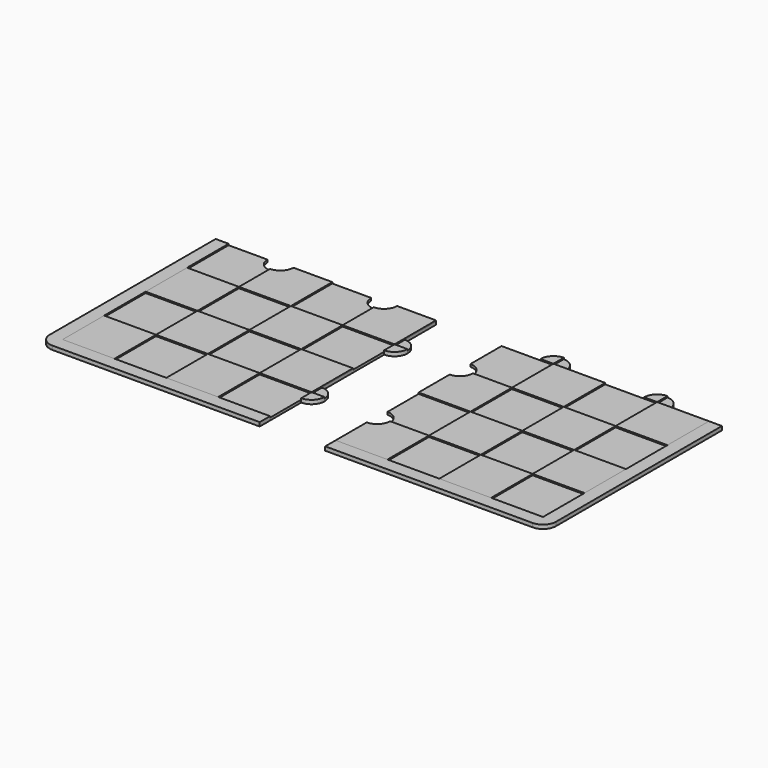
from build123d import *

# Parameters (mm, degrees)
F0_W      = 40
F0_H      = 40
F1_DEPTH  = 2
F3_DEPTH  = 2
F4_DEPTH  = 5
F2_W      = 40
F2_H      = 40
F5_DEPTH  = 1
F6_DEPTH  = 2
F7_DEPTH  = 3
F8_DEPTH  = 4
F9_DEPTH  = 3
F10_DEPTH = 3
F11_DEPTH = 3
F12_DEPTH = 2


with BuildPart() as f1:
    # F0 (on Top) → F1 (new body)
    with BuildSketch(Plane.XY):
        with BuildLine():
            Line((-100, -20), (-60, -20))
            Line((-60, -20), (-60, 10))
            ThreePointArc((-60, 10), (-67.0710678119, 12.9289321881), (-70, 20))
            Line((-70, 20), (-100, 20))
            Line((-100, 20), (-100, -20))
        make_face()
        with BuildLine():
            ThreePointArc((-70, 20), (-67.0710678119, 12.9289321881), (-60, 10))
            Line((-60, 10), (-60, 20))
            Line((-60, 20), (-70, 20))
        make_face()
        with BuildLine():
            ThreePointArc((-60, 10), (-52.9289321881, 12.9289321881), (-50, 20))
            Line((-50, 20), (-60, 20))
            Line((-60, 20), (-60, 10))
        make_face()
        with BuildLine():
            Line((-60, -20), (-20, -20))
            Line((-20, -20), (-20, 20))
            Line((-20, 20), (-50, 20))
            ThreePointArc((-50, 20), (-52.9289321881, 12.9289321881), (-60, 10))
            Line((-60, 10), (-60, -20))
        make_face()
        with BuildLine():
            Line((-20, -20), (20, -20))
            Line((20, -20), (20, 10))
            ThreePointArc((20, 10), (12.9289321881, 12.9289321881), (10, 20))
            Line((10, 20), (-20, 20))
            Line((-20, 20), (-20, -20))
        make_face()
        with BuildLine():
            ThreePointArc((10, 20), (12.9289321881, 12.9289321881), (20, 10))
            Line((20, 10), (20, 20))
            Line((20, 20), (10, 20))
        make_face()
        with BuildLine():
            Line((20, 20), (20, 10))
            ThreePointArc((20, 10), (27.0710678119, 12.9289321881), (30, 20))
            Line((30, 20), (20, 20))
        make_face()
        with BuildLine():
            Line((20, 10), (20, -20))
            Line((20, -20), (50, -20))
            ThreePointArc((50, -20), (52.9289321881, -12.9289321881), (60, -10))
            Line((60, -10), (60, 20))
            Line((60, 20), (30, 20))
            ThreePointArc((30, 20), (27.0710678119, 12.9289321881), (20, 10))
        make_face()
        with BuildLine():
            ThreePointArc((60, -10), (52.9289321881, -12.9289321881), (50, -20))
            Line((50, -20), (60, -20))
            Line((60, -20), (60, -10))
        make_face()
        with BuildLine():
            Line((60, -20), (50, -20))
            ThreePointArc((50, -20), (52.9289321881, -27.0710678119), (60, -30))
            Line((60, -30), (60, -20))
        make_face()
        with BuildLine():
            Line((50, -20), (20, -20))
            Line((20, -20), (20, -60))
            Line((20, -60), (60, -60))
            Line((60, -60), (60, -30))
            ThreePointArc((60, -30), (52.9289321881, -27.0710678119), (50, -20))
        make_face()
        with Locations((0, -40)):
            Rectangle(F0_W, F0_H)
        with Locations((-40, -40)):
            Rectangle(F0_W, F0_H)
        with Locations((-80, -40)):
            Rectangle(F0_W, F0_H)
        with Locations((-80, -80)):
            Rectangle(F0_W, F0_H)
        with BuildLine():
            Line((-60, -140), (-60, -100))
            Line((-60, -100), (-100, -100))
            Line((-100, -100), (-100, -130))
            ThreePointArc((-100, -130), (-92.9289321881, -132.9289321881), (-90, -140))
            Line((-90, -140), (-60, -140))
        make_face()
        with Locations((-40, -120)):
            Rectangle(F0_W, F0_H)
        with Locations((-40, -80)):
            Rectangle(F0_W, F0_H)
        with Locations((0, -80)):
            Rectangle(F0_W, F0_H)
        with Locations((0, -120)):
            Rectangle(F0_W, F0_H)
        with BuildLine():
            Line((50, -100), (20, -100))
            Line((20, -100), (20, -140))
            Line((20, -140), (60, -140))
            Line((60, -140), (60, -110))
            ThreePointArc((60, -110), (52.9289321881, -107.0710678119), (50, -100))
        make_face()
        with BuildLine():
            Line((60, -60), (20, -60))
            Line((20, -60), (20, -100))
            Line((20, -100), (50, -100))
            ThreePointArc((50, -100), (52.9289321881, -92.9289321881), (60, -90))
            Line((60, -90), (60, -60))
        make_face()
        with BuildLine():
            Line((60, -100), (60, -90))
            ThreePointArc((60, -90), (52.9289321881, -92.9289321881), (50, -100))
            Line((50, -100), (60, -100))
        make_face()
        with BuildLine():
            Line((60, -100), (50, -100))
            ThreePointArc((50, -100), (52.9289321881, -107.0710678119), (60, -110))
            Line((60, -110), (60, -100))
        make_face()
        with BuildLine():
            ThreePointArc((-90, -140), (-92.9289321881, -132.9289321881), (-100, -130))
            Line((-100, -130), (-100, -140))
            Line((-100, -140), (-90, -140))
        make_face()
    extrude(amount=F1_DEPTH)

    # F0 (on Top) → F3 (join)
    with BuildSketch(Plane.XY):
        with BuildLine():
            ThreePointArc((70, -100), (67.0710678119, -92.9289321881), (60, -90))
            Line((60, -90), (60, -100))
            Line((60, -100), (70, -100))
        make_face()
        with BuildLine():
            Line((60, -10), (60, -20))
            Line((60, -20), (70, -20))
            ThreePointArc((70, -20), (67.0710678119, -12.9289321881), (60, -10))
        make_face()
    extrude(amount=F3_DEPTH)

    # F0 (on Top) → F4 (cut)
    with BuildSketch(Plane.XY):
        with BuildLine():
            ThreePointArc((-70, 20), (-67.0710678119, 12.9289321881), (-60, 10))
            Line((-60, 10), (-60, 20))
            Line((-60, 20), (-70, 20))
        make_face()
        with BuildLine():
            ThreePointArc((-60, 10), (-52.9289321881, 12.9289321881), (-50, 20))
            Line((-50, 20), (-60, 20))
            Line((-60, 20), (-60, 10))
        make_face()
        with BuildLine():
            ThreePointArc((10, 20), (12.9289321881, 12.9289321881), (20, 10))
            Line((20, 10), (20, 20))
            Line((20, 20), (10, 20))
        make_face()
        with BuildLine():
            Line((20, 20), (20, 10))
            ThreePointArc((20, 10), (27.0710678119, 12.9289321881), (30, 20))
            Line((30, 20), (20, 20))
        make_face()
    extrude(amount=F4_DEPTH, mode=Mode.SUBTRACT)

    # F0 (on Top) → F10 (join)
    with BuildSketch(Plane.XY):
        with BuildLine():
            Line((70, -100), (60, -100))
            Line((60, -100), (60, -110))
            ThreePointArc((60, -110), (67.0710678119, -107.0710678119), (70, -100))
        make_face()
        with BuildLine():
            Line((70, -20), (60, -20))
            Line((60, -20), (60, -30))
            ThreePointArc((60, -30), (67.0710678119, -27.0710678119), (70, -20))
        make_face()
    extrude(amount=F10_DEPTH)


with BuildPart() as f5:
    # F2 (on face) → F5 (new body)
    with BuildSketch(Plane.XY.offset(2)):
        with Locations((-80, -120)):
            Rectangle(F2_W, F2_H)
    extrude(amount=F5_DEPTH)


with BuildPart() as f5b:
    # F2 (on face) → F5, piece 2 (new body)
    with BuildSketch(Plane.XY.offset(2)):
        with Locations((0, -120)):
            Rectangle(F2_W, F2_H)
    extrude(amount=F5_DEPTH)


with BuildPart() as f5c:
    # F2 (on face) → F5, piece 3 (new body)
    with BuildSketch(Plane.XY.offset(2)):
        with Locations((-40, -80)):
            Rectangle(F2_W, F2_H)
    extrude(amount=F5_DEPTH)


with BuildPart() as f5d:
    # F2 (on face) → F5, piece 4 (new body)
    with BuildSketch(Plane.XY.offset(2)):
        with Locations((40, -80)):
            Rectangle(F2_W, F2_H)
    extrude(amount=F5_DEPTH)


with BuildPart() as f5e:
    # F2 (on face) → F5, piece 5 (new body)
    with BuildSketch(Plane.XY.offset(2)):
        with Locations((-80, -40)):
            Rectangle(F2_W, F2_H)
    extrude(amount=F5_DEPTH)


with BuildPart() as f5f:
    # F2 (on face) → F5, piece 6 (new body)
    with BuildSketch(Plane.XY.offset(2)):
        with Locations((0, -40)):
            Rectangle(F2_W, F2_H)
    extrude(amount=F5_DEPTH)


with BuildPart() as f5g:
    # F2 (on face) → F5, piece 7 (new body)
    with BuildSketch(Plane.XY.offset(2)):
        with BuildLine():
            Line((60, -20), (60, 20))
            Line((60, 20), (30, 20))
            ThreePointArc((30, 20), (27.0710678119, 12.9289321881), (20, 10))
            Line((20, 10), (20, -20))
            Line((20, -20), (60, -20))
        make_face()
    extrude(amount=F5_DEPTH)


with BuildPart() as f5h:
    # F2 (on face) → F5, piece 8 (new body)
    with BuildSketch(Plane.XY.offset(2)):
        with BuildLine():
            Line((-60, -20), (-20, -20))
            Line((-20, -20), (-20, 20))
            Line((-20, 20), (-50, 20))
            ThreePointArc((-50, 20), (-52.9289321881, 12.9289321881), (-60, 10))
            Line((-60, 10), (-60, -20))
        make_face()
    extrude(amount=F5_DEPTH)


with BuildPart() as f6:
    # F0 (on Top) → F6 (new body)
    with BuildSketch(Plane.XY):
        with BuildLine():
            Line((150.5487942696, -140), (150.5487942696, -100))
            Line((150.5487942696, -100), (120.5487942696, -100))
            ThreePointArc((120.5487942696, -100), (117.6198620814, -107.0710678119), (110.5487942696, -110))
            Line((110.5487942696, -110), (110.5487942696, -140))
            Line((110.5487942696, -140), (150.5487942696, -140))
        make_face()
        with BuildLine():
            ThreePointArc((110.5487942696, -110), (117.6198620814, -107.0710678119), (120.5487942696, -100))
            Line((120.5487942696, -100), (110.5487942696, -100))
            Line((110.5487942696, -100), (110.5487942696, -110))
        make_face()
        with BuildLine():
            ThreePointArc((120.5487942696, -100), (117.6198620814, -92.9289321881), (110.5487942696, -90))
            Line((110.5487942696, -90), (110.5487942696, -100))
            Line((110.5487942696, -100), (120.5487942696, -100))
        make_face()
        with BuildLine():
            Line((150.5487942696, -100), (150.5487942696, -60))
            Line((150.5487942696, -60), (110.5487942696, -60))
            Line((110.5487942696, -60), (110.5487942696, -90))
            ThreePointArc((110.5487942696, -90), (117.6198620814, -92.9289321881), (120.5487942696, -100))
            Line((120.5487942696, -100), (150.5487942696, -100))
        make_face()
        with BuildLine():
            Line((150.5487942696, -20), (120.5487942696, -20))
            ThreePointArc((120.5487942696, -20), (117.6198620814, -27.0710678119), (110.5487942696, -30))
            Line((110.5487942696, -30), (110.5487942696, -60))
            Line((110.5487942696, -60), (150.5487942696, -60))
            Line((150.5487942696, -60), (150.5487942696, -20))
        make_face()
        with BuildLine():
            Line((120.5487942696, -20), (110.5487942696, -20))
            Line((110.5487942696, -20), (110.5487942696, -30))
            ThreePointArc((110.5487942696, -30), (117.6198620814, -27.0710678119), (120.5487942696, -20))
        make_face()
        with BuildLine():
            ThreePointArc((120.5487942696, -20), (117.6198620814, -12.9289321881), (110.5487942696, -10))
            Line((110.5487942696, -10), (110.5487942696, -20))
            Line((110.5487942696, -20), (120.5487942696, -20))
        make_face()
        with BuildLine():
            Line((140.5487942696, 20), (110.5487942696, 20))
            Line((110.5487942696, 20), (110.5487942696, -10))
            ThreePointArc((110.5487942696, -10), (117.6198620814, -12.9289321881), (120.5487942696, -20))
            Line((120.5487942696, -20), (150.5487942696, -20))
            Line((150.5487942696, -20), (150.5487942696, 10))
            ThreePointArc((150.5487942696, 10), (143.4777264577, 12.9289321881), (140.5487942696, 20))
        make_face()
        with BuildLine():
            Line((150.5487942696, 20), (140.5487942696, 20))
            ThreePointArc((140.5487942696, 20), (143.4777264577, 12.9289321881), (150.5487942696, 10))
            Line((150.5487942696, 10), (150.5487942696, 20))
        make_face()
        with BuildLine():
            Line((160.5487942696, 20), (150.5487942696, 20))
            Line((150.5487942696, 20), (150.5487942696, 10))
            ThreePointArc((150.5487942696, 10), (157.6198620814, 12.9289321881), (160.5487942696, 20))
        make_face()
        with BuildLine():
            ThreePointArc((160.5487942696, 20), (157.6198620814, 12.9289321881), (150.5487942696, 10))
            Line((150.5487942696, 10), (150.5487942696, -20))
            Line((150.5487942696, -20), (190.5487942696, -20))
            Line((190.5487942696, -20), (190.5487942696, 20))
            Line((190.5487942696, 20), (160.5487942696, 20))
        make_face()
        with BuildLine():
            Line((220.5487942696, 20), (190.5487942696, 20))
            Line((190.5487942696, 20), (190.5487942696, -20))
            Line((190.5487942696, -20), (230.5487942696, -20))
            Line((230.5487942696, -20), (230.5487942696, 10))
            ThreePointArc((230.5487942696, 10), (223.4777264577, 12.9289321881), (220.5487942696, 20))
        make_face()
        with BuildLine():
            Line((230.5487942696, 20), (220.5487942696, 20))
            ThreePointArc((220.5487942696, 20), (223.4777264577, 12.9289321881), (230.5487942696, 10))
            Line((230.5487942696, 10), (230.5487942696, 20))
        make_face()
        with BuildLine():
            Line((240.5487942696, 20), (230.5487942696, 20))
            Line((230.5487942696, 20), (230.5487942696, 10))
            ThreePointArc((230.5487942696, 10), (237.6198620814, 12.9289321881), (240.5487942696, 20))
        make_face()
        with BuildLine():
            Line((230.5487942696, 10), (230.5487942696, -20))
            Line((230.5487942696, -20), (270.5487942696, -20))
            Line((270.5487942696, -20), (270.5487942696, 20))
            Line((270.5487942696, 20), (240.5487942696, 20))
            ThreePointArc((240.5487942696, 20), (237.6198620814, 12.9289321881), (230.5487942696, 10))
        make_face()
        with Locations((250.5487942696, -40)):
            Rectangle(F0_W, F0_H)
        with Locations((210.5487942696, -40)):
            Rectangle(F0_W, F0_H)
        with Locations((170.5487942696, -40)):
            Rectangle(F0_W, F0_H)
        with Locations((170.5487942696, -80)):
            Rectangle(F0_W, F0_H)
        with Locations((210.5487942696, -80)):
            Rectangle(F0_W, F0_H)
        with Locations((250.5487942696, -80)):
            Rectangle(F0_W, F0_H)
        with BuildLine():
            Line((270.5487942696, -100), (230.5487942696, -100))
            Line((230.5487942696, -100), (230.5487942696, -140))
            Line((230.5487942696, -140), (260.5487942696, -140))
            ThreePointArc((260.5487942696, -140), (263.4777264577, -132.9289321881), (270.5487942696, -130))
            Line((270.5487942696, -130), (270.5487942696, -100))
        make_face()
        with Locations((210.5487942696, -120)):
            Rectangle(F0_W, F0_H)
        with Locations((170.5487942696, -120)):
            Rectangle(F0_W, F0_H)
        with BuildLine():
            ThreePointArc((270.5487942696, -130), (263.4777264577, -132.9289321881), (260.5487942696, -140))
            Line((260.5487942696, -140), (270.5487942696, -140))
            Line((270.5487942696, -140), (270.5487942696, -130))
        make_face()
    extrude(amount=F6_DEPTH)

    # F0 (on Top) → F7 (join)
    with BuildSketch(Plane.XY):
        with BuildLine():
            ThreePointArc((150.5487942696, 30), (143.4777264577, 27.0710678119), (140.5487942696, 20))
            Line((140.5487942696, 20), (150.5487942696, 20))
            Line((150.5487942696, 20), (150.5487942696, 30))
        make_face()
        with BuildLine():
            ThreePointArc((230.5487942696, 30), (223.4777264577, 27.0710678119), (220.5487942696, 20))
            Line((220.5487942696, 20), (230.5487942696, 20))
            Line((230.5487942696, 20), (230.5487942696, 30))
        make_face()
    extrude(amount=F7_DEPTH)

    # F0 (on Top) → F8 (cut)
    with BuildSketch(Plane.XY):
        with BuildLine():
            ThreePointArc((120.5487942696, -100), (117.6198620814, -92.9289321881), (110.5487942696, -90))
            Line((110.5487942696, -90), (110.5487942696, -100))
            Line((110.5487942696, -100), (120.5487942696, -100))
        make_face()
        with BuildLine():
            ThreePointArc((110.5487942696, -110), (117.6198620814, -107.0710678119), (120.5487942696, -100))
            Line((120.5487942696, -100), (110.5487942696, -100))
            Line((110.5487942696, -100), (110.5487942696, -110))
        make_face()
        with BuildLine():
            ThreePointArc((120.5487942696, -20), (117.6198620814, -12.9289321881), (110.5487942696, -10))
            Line((110.5487942696, -10), (110.5487942696, -20))
            Line((110.5487942696, -20), (120.5487942696, -20))
        make_face()
        with BuildLine():
            Line((120.5487942696, -20), (110.5487942696, -20))
            Line((110.5487942696, -20), (110.5487942696, -30))
            ThreePointArc((110.5487942696, -30), (117.6198620814, -27.0710678119), (120.5487942696, -20))
        make_face()
    extrude(amount=F8_DEPTH, mode=Mode.SUBTRACT)


with BuildPart() as f9:
    # F0 (on Top) → F9 (new body)
    with BuildSketch(Plane.XY):
        with BuildLine():
            Line((-100, -60), (-100, -20))
            Line((-100, -20), (-100, 20))
            Line((-100, 20), (-110, 20))
            Line((-110, 20), (-110, -140))
            ThreePointArc((-110, -140), (-107.0710678119, -132.9289321881), (-100, -130))
            Line((-100, -130), (-100, -100))
            Line((-100, -100), (-100, -60))
        make_face()
        Polygon((-100, -140), (-110, -140), (-100, -150), align=None)
        with BuildLine():
            ThreePointArc((-100, -150), (-92.9289321881, -147.0710678119), (-90, -140))
            Line((-90, -140), (-100, -140))
            Line((-100, -140), (-100, -150))
        make_face()
        with BuildLine():
            Line((60, -140), (20, -140))
            Line((20, -140), (-20, -140))
            Line((-20, -140), (-60, -140))
            Line((-60, -140), (-90, -140))
            ThreePointArc((-90, -140), (-92.9289321881, -147.0710678119), (-100, -150))
            Line((-100, -150), (60, -150))
            Line((60, -150), (60, -140))
        make_face()
        with BuildLine():
            ThreePointArc((-100, -130), (-107.0710678119, -132.9289321881), (-110, -140))
            Line((-110, -140), (-100, -140))
            Line((-100, -140), (-100, -130))
        make_face()
        with BuildLine():
            Line((-100, -150), (-110, -140))
            ThreePointArc((-110, -140), (-107.0710678119, -147.0710678119), (-100, -150))
        make_face()
    extrude(amount=F9_DEPTH)


with BuildPart() as f9b:
    # F0 (on Top) → F9, piece 2 (new body)
    with BuildSketch(Plane.XY):
        with BuildLine():
            Line((190.5487942696, -140), (150.5487942696, -140))
            Line((150.5487942696, -140), (110.5487942696, -140))
            Line((110.5487942696, -140), (110.5487942696, -150))
            Line((110.5487942696, -150), (270.5487942696, -150))
            ThreePointArc((270.5487942696, -150), (263.4777264577, -147.0710678119), (260.5487942696, -140))
            Line((260.5487942696, -140), (230.5487942696, -140))
            Line((230.5487942696, -140), (190.5487942696, -140))
        make_face()
        Polygon((270.5487942696, -140), (270.5487942696, -150), (280.5487942696, -140), align=None)
        with BuildLine():
            Line((270.5487942696, 20), (270.5487942696, -20))
            Line((270.5487942696, -20), (270.5487942696, -60))
            Line((270.5487942696, -60), (270.5487942696, -100))
            Line((270.5487942696, -100), (270.5487942696, -130))
            ThreePointArc((270.5487942696, -130), (277.6198620814, -132.9289321881), (280.5487942696, -140))
            Line((280.5487942696, -140), (280.5487942696, 20))
            Line((280.5487942696, 20), (270.5487942696, 20))
        make_face()
        with BuildLine():
            ThreePointArc((260.5487942696, -140), (263.4777264577, -147.0710678119), (270.5487942696, -150))
            Line((270.5487942696, -150), (270.5487942696, -140))
            Line((270.5487942696, -140), (260.5487942696, -140))
        make_face()
        with BuildLine():
            ThreePointArc((280.5487942696, -140), (277.6198620814, -132.9289321881), (270.5487942696, -130))
            Line((270.5487942696, -130), (270.5487942696, -140))
            Line((270.5487942696, -140), (280.5487942696, -140))
        make_face()
        with BuildLine():
            Line((280.5487942696, -140), (270.5487942696, -150))
            ThreePointArc((270.5487942696, -150), (277.6198620814, -147.0710678119), (280.5487942696, -140))
        make_face()
    extrude(amount=F9_DEPTH)


with BuildPart() as f11:
    # F0 (on Top) → F11 (new body)
    with BuildSketch(Plane.XY):
        with BuildLine():
            Line((150.5487942696, -20), (120.5487942696, -20))
            ThreePointArc((120.5487942696, -20), (117.6198620814, -27.0710678119), (110.5487942696, -30))
            Line((110.5487942696, -30), (110.5487942696, -60))
            Line((110.5487942696, -60), (150.5487942696, -60))
            Line((150.5487942696, -60), (150.5487942696, -20))
        make_face()
    extrude(amount=F11_DEPTH)


with BuildPart() as f11b:
    # F0 (on Top) → F11, piece 2 (new body)
    with BuildSketch(Plane.XY):
        with BuildLine():
            Line((150.5487942696, -140), (150.5487942696, -100))
            Line((150.5487942696, -100), (120.5487942696, -100))
            ThreePointArc((120.5487942696, -100), (117.6198620814, -107.0710678119), (110.5487942696, -110))
            Line((110.5487942696, -110), (110.5487942696, -140))
            Line((110.5487942696, -140), (150.5487942696, -140))
        make_face()
    extrude(amount=F11_DEPTH)


with BuildPart() as f11c:
    # F0 (on Top) → F11, piece 3 (new body)
    with BuildSketch(Plane.XY):
        with Locations((170.5487942696, -80)):
            Rectangle(F0_W, F0_H)
    extrude(amount=F11_DEPTH)


with BuildPart() as f11d:
    # F0 (on Top) → F11, piece 4 (new body)
    with BuildSketch(Plane.XY):
        with BuildLine():
            ThreePointArc((160.5487942696, 20), (157.6198620814, 12.9289321881), (150.5487942696, 10))
            Line((150.5487942696, 10), (150.5487942696, -20))
            Line((150.5487942696, -20), (190.5487942696, -20))
            Line((190.5487942696, -20), (190.5487942696, 20))
            Line((190.5487942696, 20), (160.5487942696, 20))
        make_face()
        with BuildLine():
            Line((160.5487942696, 20), (150.5487942696, 20))
            Line((150.5487942696, 20), (150.5487942696, 10))
            ThreePointArc((150.5487942696, 10), (157.6198620814, 12.9289321881), (160.5487942696, 20))
        make_face()
    extrude(amount=F11_DEPTH)


with BuildPart() as f11e:
    # F0 (on Top) → F11, piece 5 (new body)
    with BuildSketch(Plane.XY):
        with Locations((210.5487942696, -40)):
            Rectangle(F0_W, F0_H)
    extrude(amount=F11_DEPTH)


with BuildPart() as f11f:
    # F0 (on Top) → F11, piece 6 (new body)
    with BuildSketch(Plane.XY):
        with Locations((210.5487942696, -120)):
            Rectangle(F0_W, F0_H)
    extrude(amount=F11_DEPTH)


with BuildPart() as f11g:
    # F0 (on Top) → F11, piece 7 (new body)
    with BuildSketch(Plane.XY):
        with Locations((250.5487942696, -80)):
            Rectangle(F0_W, F0_H)
    extrude(amount=F11_DEPTH)


with BuildPart() as f11h:
    # F0 (on Top) → F11, piece 8 (new body)
    with BuildSketch(Plane.XY):
        with BuildLine():
            Line((230.5487942696, 10), (230.5487942696, -20))
            Line((230.5487942696, -20), (270.5487942696, -20))
            Line((270.5487942696, -20), (270.5487942696, 20))
            Line((270.5487942696, 20), (240.5487942696, 20))
            ThreePointArc((240.5487942696, 20), (237.6198620814, 12.9289321881), (230.5487942696, 10))
        make_face()
        with BuildLine():
            Line((240.5487942696, 20), (230.5487942696, 20))
            Line((230.5487942696, 20), (230.5487942696, 10))
            ThreePointArc((230.5487942696, 10), (237.6198620814, 12.9289321881), (240.5487942696, 20))
        make_face()
    extrude(amount=F11_DEPTH)


with BuildPart() as f12:
    # F0 (on Top) → F12 (new body)
    with BuildSketch(Plane.XY):
        with BuildLine():
            Line((150.5487942696, 30), (150.5487942696, 20))
            Line((150.5487942696, 20), (160.5487942696, 20))
            ThreePointArc((160.5487942696, 20), (157.6198620814, 27.0710678119), (150.5487942696, 30))
        make_face()
    extrude(amount=F12_DEPTH)


with BuildPart() as f12b:
    # F0 (on Top) → F12, piece 2 (new body)
    with BuildSketch(Plane.XY):
        with BuildLine():
            Line((230.5487942696, 30), (230.5487942696, 20))
            Line((230.5487942696, 20), (240.5487942696, 20))
            ThreePointArc((240.5487942696, 20), (237.6198620814, 27.0710678119), (230.5487942696, 30))
        make_face()
    extrude(amount=F12_DEPTH)


solid = Compound([f1.part, f5.part, f5b.part, f5c.part, f5d.part, f5e.part, f5f.part, f5g.part, f5h.part, f6.part, f9.part, f9b.part, f11.part, f11b.part, f11c.part, f11d.part, f11e.part, f11f.part, f11g.part, f11h.part, f12.part, f12b.part])
